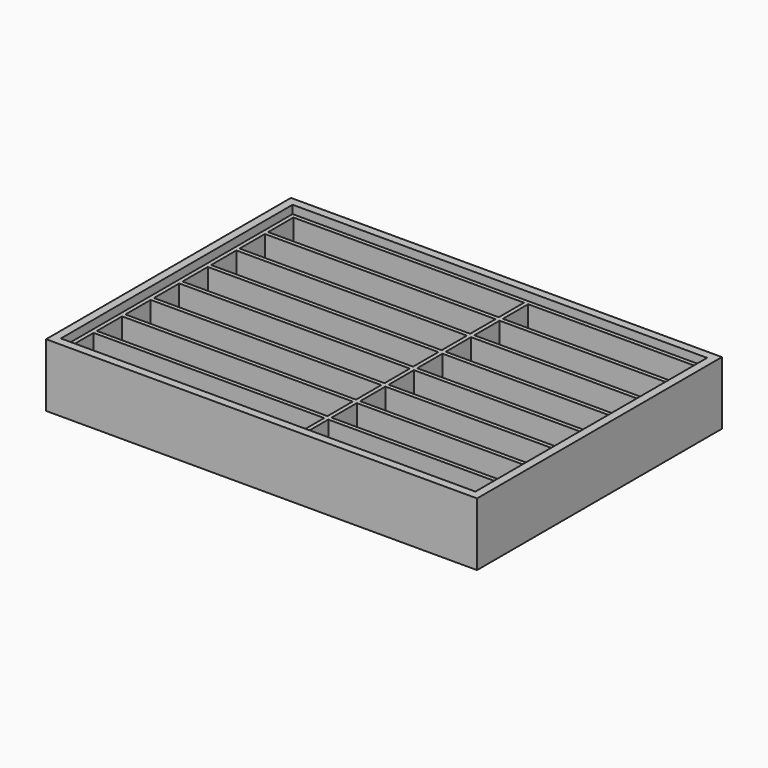
from build123d import *

# Parameters (mm, degrees)
F0_W     = 498.475
F0_H     = 354.0125
F0_W_2   = 479.425
F0_H_2   = 334.9625
F1_DEPTH = 66.675
F0_W_3   = 266.7
F0_H_3   = 36.5125
F0_W_4   = 198.4375
F2_DEPTH = 57.15
F3_W     = 498.475
F3_H     = 354.0125
F4_DEPTH = 6.35


with BuildPart() as f1:
    # F0 (on Top) → F1 (new body)
    with BuildSketch(Plane.XY):
        with Locations((-10.8039700516, 18.2372602986)):
            Rectangle(F0_W, F0_H)
        with Locations((-10.8039700516, 18.2372602986)):
            Rectangle(F0_W_2, F0_H_2, mode=Mode.SUBTRACT)
    extrude(amount=F1_DEPTH)

    # F3 (on face) → F4 (join)
    with BuildSketch(Plane.XY):
        with Locations((-10.8039700516, 18.2372602986)):
            Rectangle(F3_W, F3_H)
    extrude(amount=-F4_DEPTH)


with BuildPart() as f2:
    # F0 (on Top) → F2 (new body)
    with BuildSketch(Plane.XY):
        with Locations((-10.8039700516, 18.2372602986)):
            Rectangle(F0_W_2, F0_H_2)
        with Locations((-112.4039700516, -126.2252397014)):
            Rectangle(F0_W_3, F0_H_3, mode=Mode.SUBTRACT)
        with Locations((-112.4039700516, -84.9502397014)):
            Rectangle(F0_W_3, F0_H_3, mode=Mode.SUBTRACT)
        with Locations((-112.4039700516, -43.6752397014)):
            Rectangle(F0_W_3, F0_H_3, mode=Mode.SUBTRACT)
        with Locations((-112.4039700516, -2.4002397014)):
            Rectangle(F0_W_3, F0_H_3, mode=Mode.SUBTRACT)
        with Locations((124.9272799484, -126.2252397014)):
            Rectangle(F0_W_4, F0_H_3, mode=Mode.SUBTRACT)
        with Locations((124.9272799484, -84.9502397014)):
            Rectangle(F0_W_4, F0_H_3, mode=Mode.SUBTRACT)
        with Locations((124.9272799484, -43.6752397014)):
            Rectangle(F0_W_4, F0_H_3, mode=Mode.SUBTRACT)
        with Locations((124.9272799484, -2.4002397014)):
            Rectangle(F0_W_4, F0_H_3, mode=Mode.SUBTRACT)
        with Locations((-112.4039700516, 38.8747602986)):
            Rectangle(F0_W_3, F0_H_3, mode=Mode.SUBTRACT)
        with Locations((-112.4039700516, 80.1497602986)):
            Rectangle(F0_W_3, F0_H_3, mode=Mode.SUBTRACT)
        with Locations((-112.4039700516, 121.4247602986)):
            Rectangle(F0_W_3, F0_H_3, mode=Mode.SUBTRACT)
        with Locations((-112.4039700516, 162.6997602986)):
            Rectangle(F0_W_3, F0_H_3, mode=Mode.SUBTRACT)
        with Locations((124.9272799484, 38.8747602986)):
            Rectangle(F0_W_4, F0_H_3, mode=Mode.SUBTRACT)
        with Locations((124.9272799484, 80.1497602986)):
            Rectangle(F0_W_4, F0_H_3, mode=Mode.SUBTRACT)
        with Locations((124.9272799484, 121.4247602986)):
            Rectangle(F0_W_4, F0_H_3, mode=Mode.SUBTRACT)
        with Locations((124.9272799484, 162.6997602986)):
            Rectangle(F0_W_4, F0_H_3, mode=Mode.SUBTRACT)
    extrude(amount=F2_DEPTH)


solid = Compound([f1.part, f2.part])
